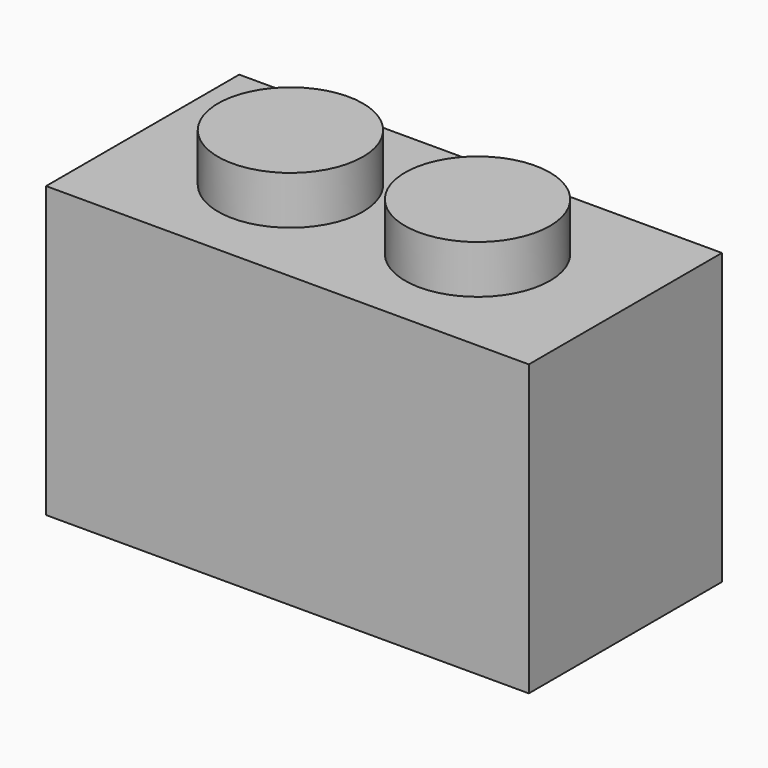
from build123d import *

# Parameters (mm, degrees)
F0_W     = 16
F0_H     = 8
F0_W_2   = 12.8
F0_H_2   = 4.8
F1_DEPTH = 9.6
F2_DEPTH = 8
F3_R     = 1.6
F4_DEPTH = 3.2
F5_R     = 2.4
F6_DEPTH = 1.6


# Not quite as in the source:
# - the program builds the solid bodies; features that only make, move or delete a surface that nothing else refers to are left out


with BuildPart() as f1:
    # F0 (on Top) → F1 (new body)
    with BuildSketch(Plane.XY):
        Rectangle(F0_W, F0_H)
        Rectangle(F0_W_2, F0_H_2, mode=Mode.SUBTRACT)
        Rectangle(F0_W_2, F0_H_2)
    extrude(amount=F1_DEPTH)

    # F0 (on Top) → F2 (cut)
    with BuildSketch(Plane.XY):
        Rectangle(F0_W_2, F0_H_2)
    extrude(amount=F2_DEPTH, mode=Mode.SUBTRACT)

    # F3 (on face) → F4 (cut)
    with BuildSketch(Plane.XY.offset(9.6)):
        with Locations((-3.1, 0)):
            Circle(F3_R)
        with Locations((3.1, 0)):
            Circle(F3_R)
    extrude(amount=-F4_DEPTH, mode=Mode.SUBTRACT)


with BuildPart() as f6:
    # F5 (on face) → F6 (new body)
    with BuildSketch(Plane.XY.offset(9.6)):
        with Locations((-3.1, 0)):
            Circle(F5_R)
    extrude(amount=F6_DEPTH)


with BuildPart() as f6b:
    # F5 (on face) → F6, piece 2 (new body)
    with BuildSketch(Plane.XY.offset(9.6)):
        with Locations((3.1, 0)):
            Circle(F5_R)
    extrude(amount=F6_DEPTH)


solid = Compound([f1.part, f6.part, f6b.part])
